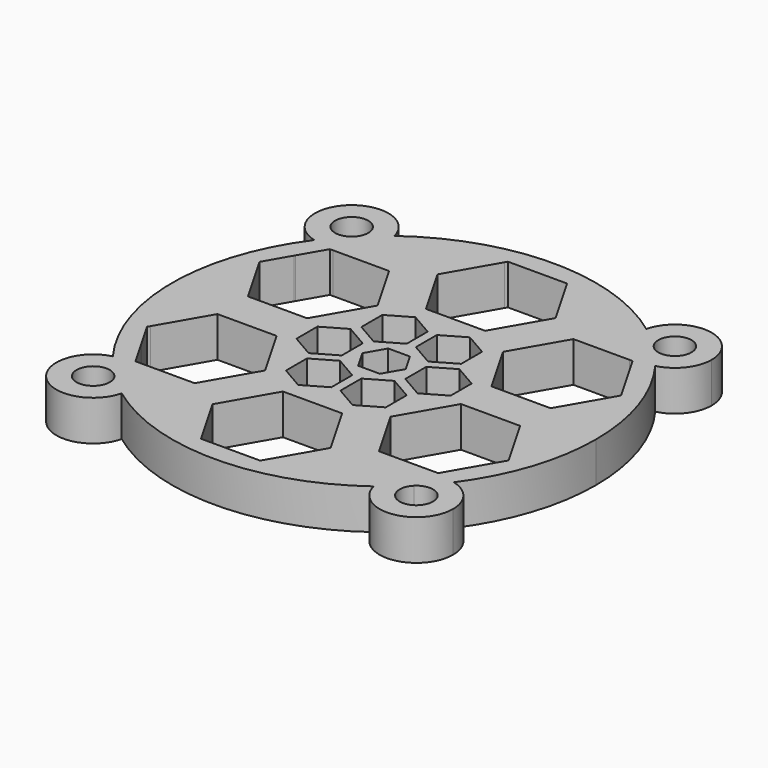
from build123d import *

# Parameters (mm, degrees)
F1_DEPTH = 4


# Not quite as in the source:
# - ends of sketch curves that miss each other by under 0.0002 mm in the source are joined


with BuildPart() as f1:
    # F0 (on Top) → F1 (new body)
    with BuildSketch(Plane.XY):
        with BuildLine():
            ThreePointArc((-14.8832723697, 14.8832737265), (-15.9503966088, 13.7334803044), (-16.9289242157, 12.5074041331))
            ThreePointArc((-16.9289242157, 12.5074041331), (-15.0725488028, 12.533313309), (-13.4690596421, 13.4690608552))
            ThreePointArc((-13.4690596421, 13.4690608552), (-12.6778389857, 14.6532061326), (-12.3999992371, 16.0500007629))
            ThreePointArc((-12.3999992371, 16.0500007629), (-12.4269495545, 16.4927320562), (-12.5074025236, 16.9289254048))
            ThreePointArc((-12.5074025236, 16.9289254048), (-13.7334788191, 15.9503978876), (-14.8832723697, 14.8832737265))
        make_face()
        with BuildLine():
            ThreePointArc((12.5074038131, 16.9289244521), (8.016e-07, 21.0481265971), (-12.5074025236, 16.9289254048))
            ThreePointArc((-12.5074025236, 16.9289254048), (-12.4269495545, 16.4927320562), (-12.3999992371, 16.0500007629))
            ThreePointArc((-12.3999992371, 16.0500007629), (-12.6778389857, 14.6532061326), (-13.4690596421, 13.4690608552))
            ThreePointArc((-13.4690596421, 13.4690608552), (-8.6931773802, 16.9487401861), (-3.0807040231, 18.7973506001))
            Line((-3.0807040231, 18.7973506001), (-2.9359184337, 19.0481265971))
            Line((-2.9359184337, 19.0481265971), (3.1e-08, 19.0481265971))
            Line((3.1e-08, 19.0481265971), (2.9359184337, 19.0481265971))
            Line((2.9359184337, 19.0481265971), (3.0807040231, 18.7973506001))
            ThreePointArc((3.0807040231, 18.7973506001), (8.6931777594, 16.9487399916), (13.4690594818, 13.4690594896))
            ThreePointArc((13.4690594818, 13.4690594896), (12.5333135158, 15.0725495848), (12.5074038131, 16.9289244521))
        make_face()
        with BuildLine():
            ThreePointArc((14.8832730679, 14.8832730283), (13.7334798008, 15.9503970424), (12.5074038131, 16.9289244521))
            ThreePointArc((12.5074038131, 16.9289244521), (12.5333135158, 15.0725495848), (13.4690610077, 13.4690610155))
            ThreePointArc((13.4690610077, 13.4690610155), (15.0725495795, 12.5333135173), (16.9289244521, 12.5074038131))
            ThreePointArc((16.9289244521, 12.5074038131), (15.9503970607, 13.7334797795), (14.8832730679, 14.8832730283))
        make_face()
        with BuildLine():
            ThreePointArc((14.7389042455, -12.0663096472), (14.1214106882, -12.7834614653), (13.469060126, -13.4690588454))
            ThreePointArc((13.469060126, -13.4690588454), (15.0725499715, -12.5333118824), (16.9289254048, -12.5074025236))
            ThreePointArc((16.9289254048, -12.5074025236), (19.9918208065, -6.5841274356), (21.0481265971, 0))
            ThreePointArc((21.0481265971, 0), (19.9918205558, 6.584128197), (16.9289244521, 12.5074038131))
            ThreePointArc((16.9289244521, 12.5074038131), (15.0725495795, 12.5333135173), (13.4690610077, 13.4690610155))
            ThreePointArc((13.4690610077, 13.4690610155), (14.1212174462, 12.7836749293), (14.7385400167, 12.0667545362))
            Line((14.7385400167, 12.0667545362), (15.0280097995, 12.0667545415))
            Line((15.0280097995, 12.0667545415), (16.4635485578, 9.5803285823))
            ThreePointArc((16.4635485578, 9.5803285823), (16.496161351, 9.5240636044), (16.5285818567, 9.4676876093))
            Line((16.5285818567, 9.4676876093), (17.9639283275, 6.9815947019))
            Line((17.9639283275, 6.9815947019), (17.8192336321, 6.7309761272))
            ThreePointArc((17.8192336321, 6.7309761272), (18.7383850018, 3.4211188793), (19.0481265971, 0))
            ThreePointArc((19.0481265971, 0), (18.7384108655, -3.4209772138), (17.8193354047, -6.7307066936))
            Line((17.8193354047, -6.7307066936), (17.9639287158, -6.9811496335))
            Line((17.9639287158, -6.9811496335), (16.5521937692, -9.4263464974))
            ThreePointArc((16.5521937692, -9.4263464974), (16.4961618808, -9.5240626868), (16.4395531298, -9.6214458244))
            Line((16.4395531298, -9.6214458244), (15.0280104707, -12.0663096364))
            Line((15.0280104707, -12.0663096364), (14.7389042455, -12.0663096472))
        make_face()
        with BuildLine():
            ThreePointArc((13.469060889, -13.4690596084), (12.5333133154, -15.0725487798), (12.5074041331, -16.9289242157))
            ThreePointArc((12.5074041331, -16.9289242157), (13.7334803406, -15.9503965776), (14.8832737941, -14.8832723021))
            ThreePointArc((14.8832737941, -14.8832723021), (15.9503979188, -13.7334787829), (16.9289254048, -12.5074025236))
            ThreePointArc((16.9289254048, -12.5074025236), (15.0725499715, -12.5333118824), (13.469060889, -13.4690596084))
        make_face()
        with BuildLine():
            ThreePointArc((-12.3999992371, -16.0499992371), (-12.4269496351, -16.4927311897), (-12.5074028436, -16.9289251684))
            ThreePointArc((-12.5074028436, -16.9289251684), (8.016e-07, -21.0481265971), (12.5074041331, -16.9289242157))
            ThreePointArc((12.5074041331, -16.9289242157), (12.5333133154, -15.0725487798), (13.469060889, -13.4690596084))
            ThreePointArc((13.469060889, -13.4690596084), (8.693050972, -16.9488050215), (3.0804218918, -18.7973968365))
            Line((3.0804218918, -18.7973968365), (2.9359194933, -19.0476823647))
            Line((2.9359194933, -19.0476823647), (0.1300670867, -19.0476825208))
            ThreePointArc((0.1300670867, -19.0476825208), (1.0596e-06, -19.0481265971), (-0.1300649676, -19.0476825353))
            Line((-0.1300649676, -19.0476825353), (-2.9359173741, -19.0476826914))
            Line((-2.9359173741, -19.0476826914), (-3.0804198005, -18.7973971792))
            ThreePointArc((-3.0804198005, -18.7973971792), (-8.6930496263, -16.9488057118), (-13.4690594857, -13.4690594857))
            ThreePointArc((-13.4690594857, -13.4690594857), (-12.6778389434, -14.6532047089), (-12.3999992371, -16.0499992371))
        make_face()
        with BuildLine():
            ThreePointArc((-16.9289251684, -12.5074028436), (-15.9503974445, -13.7334793337), (-14.8832730474, -14.8832730488))
            ThreePointArc((-14.8832730474, -14.8832730488), (-13.733479333, -15.9503974452), (-12.5074028436, -16.9289251684))
            ThreePointArc((-12.5074028436, -16.9289251684), (-12.4269496351, -16.4927311897), (-12.3999992371, -16.0499992371))
            ThreePointArc((-12.3999992371, -16.0499992371), (-12.6778389434, -14.6532047089), (-13.4690594857, -13.4690594857))
            ThreePointArc((-13.4690594857, -13.4690594857), (-15.0725491692, -12.5333116813), (-16.9289251684, -12.5074028436))
        make_face()
        with BuildLine():
            ThreePointArc((-16.9289242157, 12.5074041331), (-21.0481265971, 8.016e-07), (-16.9289251684, -12.5074028436))
            ThreePointArc((-16.9289251684, -12.5074028436), (-15.0725491692, -12.5333116813), (-13.4690594857, -13.4690594857))
            ThreePointArc((-13.4690594857, -13.4690594857), (-14.1214096732, -12.7834625865), (-14.7389029031, -12.066311287))
            Line((-14.7389029031, -12.066311287), (-15.0280091282, -12.0663113084))
            Line((-15.0280091282, -12.0663113084), (-16.4395520575, -9.6214476566))
            ThreePointArc((-16.4395520575, -9.6214476566), (-16.4961608212, -9.5240645221), (-16.5521927222, -9.4263483357))
            Line((-16.5521927222, -9.4263483357), (-17.9639279391, -6.9811516321))
            Line((-17.9639279391, -6.9811516321), (-17.8193346558, -6.7307086762))
            ThreePointArc((-17.8193346558, -6.7307086762), (-19.0481265966, 0.0001418878), (-17.8192343809, 6.7309741447))
            Line((-17.8192343809, 6.7309741447), (-17.9639291042, 6.9815927033))
            Line((-17.9639291042, 6.9815927033), (-16.5285829132, 9.4676857649))
            ThreePointArc((-16.5285829132, 9.4676857649), (-16.4961624106, 9.5240617691), (-16.4635496205, 9.5803267561))
            Line((-16.4635496205, 9.5803267561), (-15.0280111419, 12.0667528696))
            Line((-15.0280111419, 12.0667528696), (-14.7385413592, 12.0667528964))
            ThreePointArc((-14.7385413592, 12.0667528964), (-14.1212178714, 12.7836744596), (-13.4690588792, 13.4690600923))
            ThreePointArc((-13.4690588792, 13.4690600923), (-15.0725488028, 12.533313309), (-16.9289242157, 12.5074041331))
        make_face()
        with BuildLine():
            ThreePointArc((-12.5074025236, 16.9289254048), (-18.6309388657, 18.630940637), (-16.9289242157, 12.5074041331))
            ThreePointArc((-16.9289242157, 12.5074041331), (-15.9503966088, 13.7334803044), (-14.8832723697, 14.8832737265))
            ThreePointArc((-14.8832723697, 14.8832737265), (-13.7334788191, 15.9503978876), (-12.5074025236, 16.9289254048))
        make_face()
        with BuildLine():
            ThreePointArc((-14.3999992371, 16.0500007629), (-14.5255980313, 15.4185730443), (-14.8832731326, 14.8832744894))
            ThreePointArc((-14.8832731326, 14.8832744894), (-17.5744004428, 16.6814284816), (-14.3999992371, 16.0500007629))
        make_face(mode=Mode.SUBTRACT)
        with BuildLine():
            ThreePointArc((19.7000007629, 16.0500007629), (16.492731569, 19.673050505), (12.5074038131, 16.9289244521))
            ThreePointArc((12.5074038131, 16.9289244521), (13.7334798008, 15.9503970424), (14.8832730679, 14.8832730283))
            ThreePointArc((14.8832730679, 14.8832730283), (15.9503970607, 13.7334797795), (16.9289244521, 12.5074038131))
            ThreePointArc((16.9289244521, 12.5074038131), (18.9249417593, 13.801175677), (19.7000007629, 16.0500007629))
        make_face()
        with BuildLine():
            ThreePointArc((17.7000007629, 16.0500007629), (16.6814284393, 14.5255995397), (14.8832745938, 14.8832745541))
            ThreePointArc((14.8832745938, 14.8832745541), (15.4185730866, 17.5744019862), (17.7000007629, 16.0500007629))
        make_face(mode=Mode.SUBTRACT)
        with BuildLine():
            ThreePointArc((14.8832737941, -14.8832723021), (13.7334803406, -15.9503965776), (12.5074041331, -16.9289242157))
            ThreePointArc((12.5074041331, -16.9289242157), (16.4927322284, -19.6730488985), (19.7000007629, -16.0499992371))
            ThreePointArc((19.7000007629, -16.0499992371), (18.9249420617, -13.8011745377), (16.9289254048, -12.5074025236))
            ThreePointArc((16.9289254048, -12.5074025236), (15.9503979188, -13.7334787829), (14.8832737941, -14.8832723021))
        make_face()
        with BuildLine():
            ThreePointArc((17.7000007629, -16.0499992371), (15.4185731106, -17.5744004703), (14.8832745571, -14.883273065))
            ThreePointArc((14.8832745571, -14.883273065), (16.6814284153, -14.5255980038), (17.7000007629, -16.0499992371))
        make_face(mode=Mode.SUBTRACT)
        with BuildLine():
            ThreePointArc((-12.5074028436, -16.9289251684), (-13.733479333, -15.9503974452), (-14.8832730474, -14.8832730488))
            ThreePointArc((-14.8832730474, -14.8832730488), (-15.9503974445, -13.7334793337), (-16.9289251684, -12.5074028436))
            ThreePointArc((-16.9289251684, -12.5074028436), (-18.6309389884, -18.6309389884), (-12.5074028436, -16.9289251684))
        make_face()
        with BuildLine():
            ThreePointArc((-14.8832730474, -14.8832730488), (-14.5255980082, -15.4185715741), (-14.3999992371, -16.0499992371))
            ThreePointArc((-14.3999992371, -16.0499992371), (-17.5744004659, -16.6814269), (-14.8832730474, -14.8832730488))
        make_face(mode=Mode.SUBTRACT)
        with BuildLine():
            ThreePointArc((-14.7389029031, -12.066311287), (-14.1214096732, -12.7834625865), (-13.4690594857, -13.4690594857))
            ThreePointArc((-13.4690594857, -13.4690594857), (-8.6930496263, -16.9488057118), (-3.0804198005, -18.7973971792))
            Line((-3.0804198005, -18.7973971792), (-5.8718360907, -13.9625229606))
            Line((-5.8718360907, -13.9625229606), (-2.9359179399, -8.8773629033))
            Line((-2.9359179399, -8.8773629033), (2.9359189275, -8.8773625766))
            Line((2.9359189275, -8.8773625766), (5.8718376441, -13.9625223073))
            Line((5.8718376441, -13.9625223073), (3.0804218918, -18.7973968365))
            ThreePointArc((3.0804218918, -18.7973968365), (8.693050972, -16.9488050215), (13.469060126, -13.4690588454))
            ThreePointArc((13.469060126, -13.4690588454), (14.1214106882, -12.7834614653), (14.7389042455, -12.0663096472))
            Line((14.7389042455, -12.0663096472), (9.1561736033, -12.0663098542))
            Line((9.1561736033, -12.0663098542), (6.220254981, -6.981150069))
            Line((6.220254981, -6.981150069), (9.1561732261, -1.8959900661))
            Line((9.1561732261, -1.8959900661), (15.0280100935, -1.8959898484))
            Line((15.0280100935, -1.8959898484), (17.8193354047, -6.7307066936))
            ThreePointArc((17.8193354047, -6.7307066936), (18.7384108655, -3.4209772138), (19.0481265971, 0))
            ThreePointArc((19.0481265971, 0), (18.7383850018, 3.4211188793), (17.8192336321, 6.7309761272))
            Line((17.8192336321, 6.7309761272), (15.028009988, 1.8964347534))
            Line((15.028009988, 1.8964347534), (9.1561731206, 1.8964346445))
            Line((9.1561731206, 1.8964346445), (6.2202545927, 6.9815944842))
            Line((6.2202545927, 6.9815944842), (9.1561729321, 12.0667544326))
            Line((9.1561729321, 12.0667544326), (14.7385400167, 12.0667545362))
            ThreePointArc((14.7385400167, 12.0667545362), (14.1212174462, 12.7836749293), (13.4690594818, 13.4690594896))
            ThreePointArc((13.4690594818, 13.4690594896), (8.6931777594, 16.9487399916), (3.0807040231, 18.7973506001))
            Line((3.0807040231, 18.7973506001), (5.8718368674, 13.9629667031))
            Line((5.8718368674, 13.9629667031), (2.9359184337, 8.877806809))
            Line((2.9359184337, 8.877806809), (-2.9359184337, 8.877806809))
            Line((-2.9359184337, 8.877806809), (-5.8718368674, 13.9629667031))
            Line((-5.8718368674, 13.9629667031), (-3.0807040231, 18.7973506001))
            ThreePointArc((-3.0807040231, 18.7973506001), (-8.6931773802, 16.9487401861), (-13.4690588792, 13.4690600923))
            ThreePointArc((-13.4690588792, 13.4690600923), (-14.1212178714, 12.7836744596), (-14.7385413592, 12.0667528964))
            Line((-14.7385413592, 12.0667528964), (-9.1561742745, 12.066753414))
            Line((-9.1561742745, 12.066753414), (-6.2202553694, 6.9815937921))
            Line((-6.2202553694, 6.9815937921), (-9.1561733316, 1.8964336259))
            Line((-9.1561733316, 1.8964336259), (-15.028010199, 1.8964330815))
            Line((-15.028010199, 1.8964330815), (-17.8192343809, 6.7309741447))
            ThreePointArc((-17.8192343809, 6.7309741447), (-19.0481265966, 0.0001418878), (-17.8193346558, -6.7307086762))
            Line((-17.8193346558, -6.7307086762), (-15.0280098826, -1.8959915203))
            Line((-15.0280098826, -1.8959915203), (-9.1561730152, -1.8959910848))
            Line((-9.1561730152, -1.8959910848), (-6.2202542043, -6.9811507611))
            Line((-6.2202542043, -6.9811507611), (-9.1561722608, -12.0663108729))
            Line((-9.1561722608, -12.0663108729), (-14.7389029031, -12.066311287))
        make_face()
        Polygon((-3.1563654489, -1.299038115), (-5.4063654369, -2.5980762415), (-7.6563654489, -1.2990381567), (-7.656365473, 1.2990380546), (-5.406365485, 2.5980761812), (-3.156365473, 1.2990380963), align=None, mode=Mode.SUBTRACT)
        Polygon((-0.4531827164, -3.3830117199), (-0.4531826923, -5.9810879312), (-2.7031826802, -7.2801260578), (-4.9531826923, -5.981087973), (-4.9531827164, -3.3830117616), (-2.7031827284, -2.0839736351), align=None, mode=Mode.SUBTRACT)
        Polygon((2.7031827325, -2.0839736049), (4.9531827446, -3.3830116897), (4.9531827687, -5.981087901), (2.7031827807, -7.2801260276), (0.4531827687, -5.9810879428), (0.4531827446, -3.3830117314), align=None, mode=Mode.SUBTRACT)
        Polygon((-2.7031827325, 2.0839736049), (-4.9531827446, 3.3830116897), (-4.9531827687, 5.981087901), (-2.7031827807, 7.2801260276), (-0.4531827687, 5.9810879428), (-0.4531827446, 3.3830117314), align=None, mode=Mode.SUBTRACT)
        Polygon((-2.1503604759, 0), (-1.075180238, 1.8622667994), (1.075180238, 1.8622667994), (2.1503604759, 0), (1.075180238, -1.8622667994), (-1.075180238, -1.8622667994), align=None, mode=Mode.SUBTRACT)
        Polygon((0.4531826923, 5.9810879312), (2.7031826802, 7.2801260578), (4.9531826923, 5.981087973), (4.9531827164, 3.3830117616), (2.7031827284, 2.0839736351), (0.4531827164, 3.3830117199), align=None, mode=Mode.SUBTRACT)
        Polygon((3.1563654489, 1.299038115), (5.4063654369, 2.5980762415), (7.6563654489, 1.2990381567), (7.656365473, -1.2990380546), (5.406365485, -2.5980761812), (3.156365473, -1.2990380963), align=None, mode=Mode.SUBTRACT)
    extrude(amount=F1_DEPTH)


solid = f1.part
